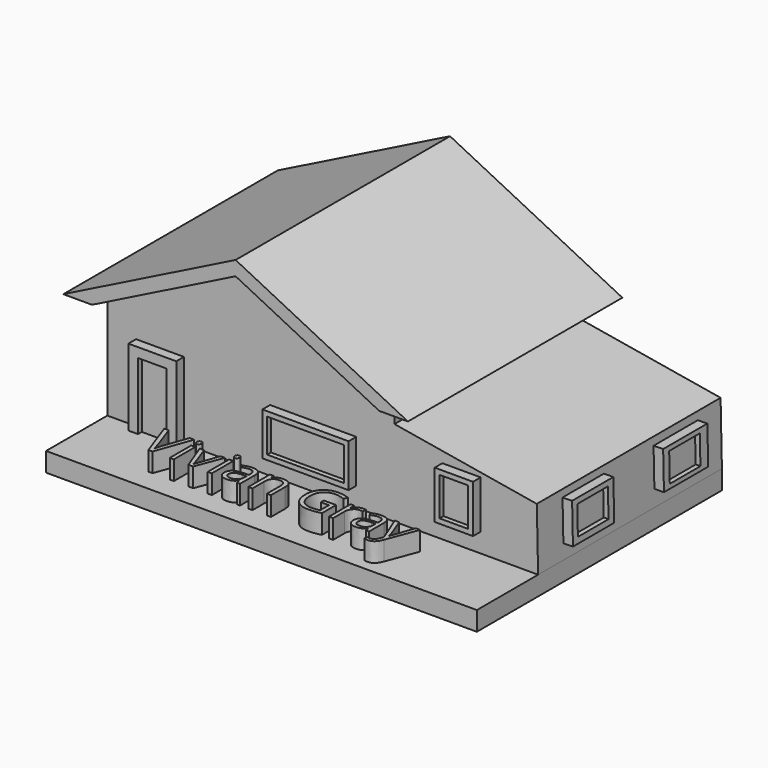
from build123d import *

# Parameters (mm, degrees)
F0_W          = 2743.2
F0_H          = 1371.6
F0_W_2        = 1219.2
F0_H_2        = 1524
F1_DEPTH      = 3657.6
F1_DEPTH_BACK = 3657.6
F0_W_3        = 914.4
F0_H_3        = 2133.6
F2_DEPTH      = 3810
F2_DEPTH_BACK = 3657.6
F0_W_4        = 2438.4
F0_H_4        = 1066.8
F0_H_5        = 1219.2
F3_DEPTH      = 3962.4
F3_DEPTH_BACK = 3657.6
F0_W_5        = 4572
F0_H_6        = 609.6
F4_DEPTH      = 6096
F4_DEPTH_BACK = 3657.6
F5_DEPTH      = 4267.2
F5_DEPTH_BACK = 4267.2
F6_TEXT_SIZE  = 1602.0165549384
F7_DEPTH      = 609.6
F8_W          = 1219.2
F8_H          = 914.4
F9_DEPTH      = 152.4
F8_W_2        = 1641.9211030006
F8_H_2        = 1275.4207849503
F8_W_3        = 1759.6059794426
F8_H_3        = 1202.120423317
F10_DEPTH     = 304.8


# Not quite as in the source:
# - Text() gives the source's letters only with a copy of the font that has no kerning and outlines rounded to 1/6400 em; it was checked with that copy


with BuildPart() as f1:
    # F0 (on Front) → F1 (new body, two sides)
    with BuildSketch(Plane.XZ) as f1_sk:
        Polygon((4572, 0), (0, 0), (-4572, 0), (-4572, -3352.8), (-3657.6, -3352.8), (-3657.6, -914.4), (-2133.6, -914.4), (-2133.6, -3352.8), (4572, -3352.8), (4572, -618.188925824), align=None)
        with Locations((1981.2, -2057.4)):
            Rectangle(F0_W, F0_H, mode=Mode.SUBTRACT)
        Polygon((-4572, 0), (0, 0), (4572, 0), (0, 2286), align=None)
        Polygon((9101.7974195729, -1381.2601979941), (4572, -618.188925824), (4572, -3352.8), (9144, -3352.8), align=None)
        with Locations((6705.6, -1981.2)):
            Rectangle(F0_W_2, F0_H_2, mode=Mode.SUBTRACT)
    extrude(amount=F1_DEPTH)
    extrude(f1_sk.sketch, amount=-F1_DEPTH_BACK)

    # F0 (on Front) → F5 (join, two sides)
    with BuildSketch(Plane.XZ) as f5_sk:
        Polygon((0, 2286), (4572, 0), (5486.4, 0), (0, 2743.2), align=None)
        Polygon((-5486.4, 0), (-4572, 0), (0, 2286), (0, 2743.2), align=None)
    extrude(amount=F5_DEPTH)
    extrude(f5_sk.sketch, amount=-F5_DEPTH_BACK)

    # F8 (on face) → F9 (join)
    with BuildSketch(Plane(origin=(9068.0751990667, 0, 194.1102951702), x_dir=(0, 1, 0), z_dir=(0.9997709725, 0, 0.0214009957))):
        with Locations((1828.8, -2437.8335979462)):
            Rectangle(F8_W, F8_H)
        with Locations((-1828.8, -2437.8335979462)):
            Rectangle(F8_W, F8_H)
    extrude(amount=F9_DEPTH)

    # F8 (on face) → F10 (join)
    with BuildSketch(Plane(origin=(9068.0751990667, 0, 194.1102951702), x_dir=(0, 1, 0), z_dir=(0.9997709725, 0, 0.0214009957))):
        with Locations((-1818.5665309429, -2447.0178484917)):
            Rectangle(F8_W_2, F8_H_2)
        with Locations((-1828.8, -2437.8335979462)):
            Rectangle(F8_W, F8_H, mode=Mode.SUBTRACT)
        with Locations((1863.3970102787, -2432.3577880859)):
            Rectangle(F8_W_3, F8_H_3)
        with Locations((1828.8, -2437.8335979462)):
            Rectangle(F8_W, F8_H, mode=Mode.SUBTRACT)
    extrude(amount=F10_DEPTH)


with BuildPart() as f2:
    # F0 (on Front) → F2 (new body, two sides)
    with BuildSketch(Plane.XZ) as f2_sk:
        with Locations((-2895.6, -2286)):
            Rectangle(F0_W_3, F0_H_3)
    extrude(amount=F2_DEPTH)
    extrude(f2_sk.sketch, amount=-F2_DEPTH_BACK)


with BuildPart() as f2b:
    # F0 (on Front) → F2, piece 2 (new body, two sides)
    with BuildSketch(Plane.XZ) as f2_2_sk:
        with Locations((1981.2, -2057.4)):
            Rectangle(F0_W_4, F0_H_4)
    extrude(amount=F2_DEPTH)
    extrude(f2_2_sk.sketch, amount=-F2_DEPTH_BACK)


with BuildPart() as f2c:
    # F0 (on Front) → F2, piece 3 (new body, two sides)
    with BuildSketch(Plane.XZ) as f2_3_sk:
        with Locations((6705.6, -1981.2)):
            Rectangle(F0_W_3, F0_H_5)
    extrude(amount=F2_DEPTH)
    extrude(f2_3_sk.sketch, amount=-F2_DEPTH_BACK)


with BuildPart() as f3:
    # F0 (on Front) → F3 (new body, two sides)
    with BuildSketch(Plane.XZ) as f3_sk:
        Polygon((-3657.6, -914.4), (-3657.6, -3352.8), (-3352.8, -3352.8), (-3352.8, -1219.2), (-2438.4, -1219.2), (-2438.4, -3352.8), (-2133.6, -3352.8), (-2133.6, -914.4), align=None)
    extrude(amount=F3_DEPTH)
    extrude(f3_sk.sketch, amount=-F3_DEPTH_BACK)


with BuildPart() as f3b:
    # F0 (on Front) → F3, piece 2 (new body, two sides)
    with BuildSketch(Plane.XZ) as f3_2_sk:
        with Locations((1981.2, -2057.4)):
            Rectangle(F0_W, F0_H)
        with Locations((1981.2, -2057.4)):
            Rectangle(F0_W_4, F0_H_4, mode=Mode.SUBTRACT)
    extrude(amount=F3_DEPTH)
    extrude(f3_2_sk.sketch, amount=-F3_DEPTH_BACK)


with BuildPart() as f3c:
    # F0 (on Front) → F3, piece 3 (new body, two sides)
    with BuildSketch(Plane.XZ) as f3_3_sk:
        with Locations((6705.6, -1981.2)):
            Rectangle(F0_W_2, F0_H_2)
        with Locations((6705.6, -1981.2)):
            Rectangle(F0_W_3, F0_H_5, mode=Mode.SUBTRACT)
    extrude(amount=F3_DEPTH)
    extrude(f3_3_sk.sketch, amount=-F3_DEPTH_BACK)


with BuildPart() as f4:
    # F0 (on Front) → F4 (new body, two sides)
    with BuildSketch(Plane.XZ) as f4_sk:
        Polygon((-3657.6, -3352.8), (-4572, -3352.8), (-4572, -3962.4), (4572, -3962.4), (4572, -3352.8), (-2133.6, -3352.8), (-2438.4, -3352.8), (-3352.8, -3352.8), align=None)
        with Locations((6858, -3657.6)):
            Rectangle(F0_W_5, F0_H_6)
    extrude(amount=F4_DEPTH)
    extrude(f4_sk.sketch, amount=-F4_DEPTH_BACK)

    # F6 (on face) → F7 (join)
    with BuildSketch(Plane.XY.offset(-3352.8)):
        with Locations((-2297.0440983772, -5380.0911903381)):
            Text('Vivian Gray', F6_TEXT_SIZE, font='Open Sans', text_align=(TextAlign.LEFT, TextAlign.BOTTOM))
    extrude(amount=F7_DEPTH)


solid = Compound([f1.part, f2.part, f2b.part, f2c.part, f3.part, f3b.part, f3c.part, f4.part])
